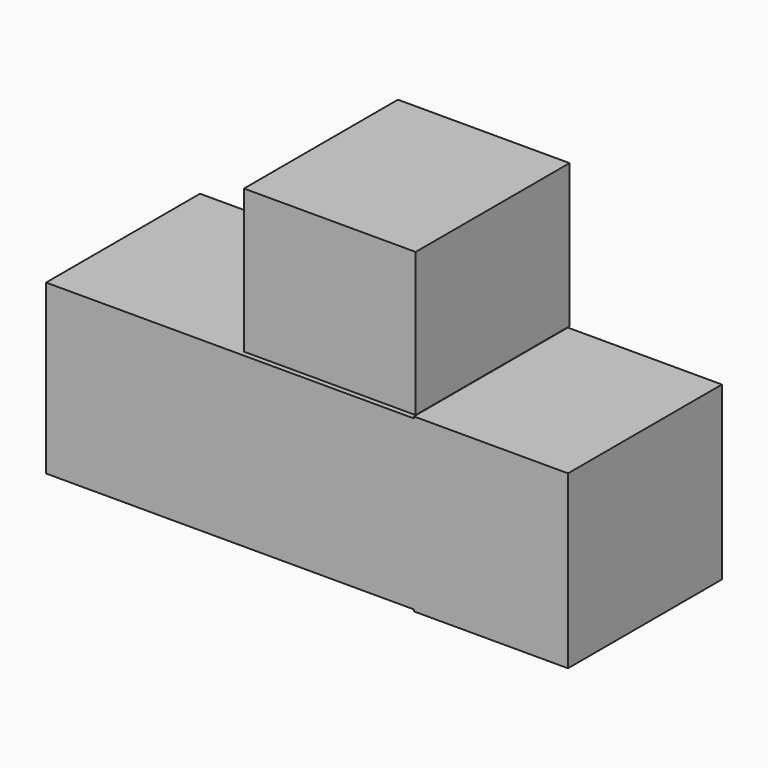
from build123d import *

# Parameters (mm, degrees)
F0_W     = 44.3958938122
F0_H     = 44.3958938122
F0_W_2   = 52.7201294899
F1_DEPTH = 50.8
F0_W_3   = 45.3208126128
F0_H_2   = 37.9214994609


# Not quite as in the source:
# - ends of sketch curves that miss each other by under 0.0002 mm in the source are joined


with BuildPart() as f1:
    # F0 (on Front) → F1 (new body)
    with BuildSketch(Plane.XZ):
        Polygon((22.1979469061, -0.92491135), (22.1979469061, -45.3208051622), (22.1979394555, -45.7832626998), (62.8941878676, -45.7832626998), (62.8941878676, -0.4624538124), (22.1979394555, -0.4624538124), align=None)
        with Locations((0, -23.1228582561)):
            Rectangle(F0_W, F0_H)
        with Locations((-48.558011651, -23.1228582561)):
            Rectangle(F0_W_2, F0_H)
    extrude(amount=F1_DEPTH)


with BuildPart() as f1b:
    # F0 (on Front) → F1, piece 2 (new body)
    with BuildSketch(Plane.XZ):
        with Locations((0, 18.9607497305)):
            Rectangle(F0_W_3, F0_H_2)
    extrude(amount=F1_DEPTH)


solid = Compound([f1.part, f1b.part])
